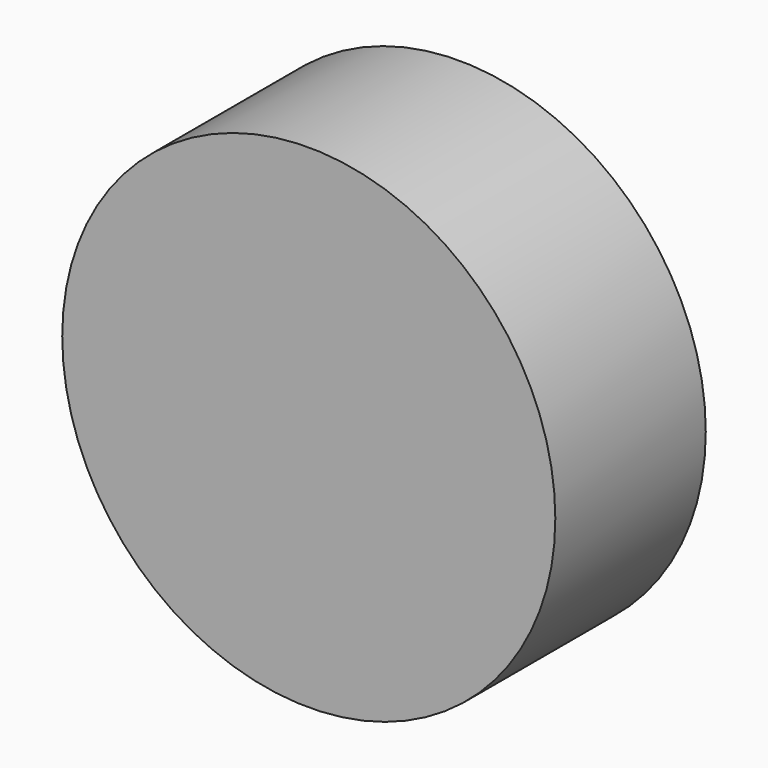
from build123d import *

# Parameters (mm, degrees)
F0_R     = 32.7728421293
F1_DEPTH = 25
F4_R     = 2.5240293439
F5_DEPTH = 25


# Not quite as in the source:
# - the program builds the solid bodies; features that only make, move or delete a surface that nothing else refers to are left out


with BuildPart() as f1:
    # F0 (on Front) → F1 (new body)
    with BuildSketch(Plane.XZ):
        with Locations((0, -2.2915014997)):
            Circle(F0_R)
    extrude(amount=F1_DEPTH)

    # F4 (on Front) → F5 (join)
    with BuildSketch(Plane.XZ):
        with Locations((0, -2.3574866354)):
            Circle(F4_R)
    extrude(amount=F5_DEPTH)


solid = f1.part
